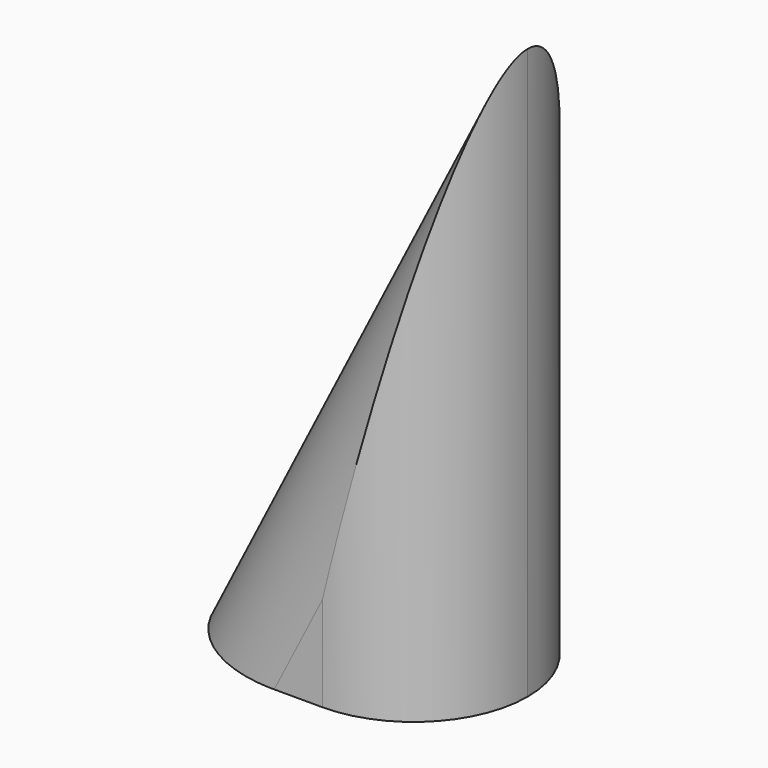
from build123d import *

# Parameters (mm, degrees)
F1_DEPTH = 10.16
F2_R     = 5.07999


# Not quite as in the source:
# - a fillet or chamfer is up to 0.001 mm smaller than in the source, because OpenCascade refuses the exact size


with BuildPart() as f1:
    # F0 (on Front) → F1 (new body)
    with BuildSketch(Plane.XZ):
        Polygon((-12.9241171581, 0), (0, 0), (0, 25.4), align=None)
    extrude(amount=F1_DEPTH)

    # F2 (radius 5.08 in the source; OpenCascade refuses exactly that, so slightly less here)
    f2_edges = [f1.edges().sort_by_distance(p)[0] for p in [
        (-6.462059, 0, 12.7),
        (-6.462059, -10.16, 12.7),
        (0, 0, 12.7),
        (0, -10.16, 12.7),
    ]]
    fillet(f2_edges, radius=F2_R)


solid = f1.part
